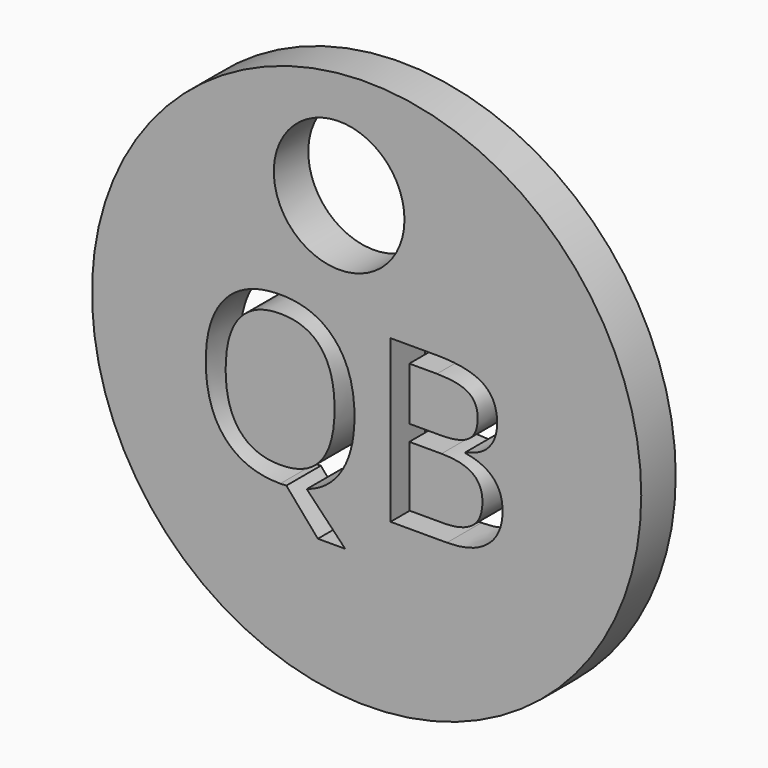
from build123d import *

# Parameters (mm, degrees)
F0_R         = 13.7039502502
F1_DEPTH     = 2.15
F2_R         = 3.2599586052
F3_DEPTH     = 2.15
F4_TEXT_SIZE = 11.3007392631
F5_DEPTH     = 2.15


# Not quite as in the source:
# - Text() gives the source's letters only with a copy of the font that has no kerning and outlines rounded to 1/6400 em; it was checked with that copy


with BuildPart() as f1:
    # F0 (on Front) → F1 (new body)
    with BuildSketch(Plane.XZ):
        with Locations((-43.4432663023, -15.2559969574)):
            Circle(F0_R)
    extrude(amount=F1_DEPTH)

    # F2 (on Front) → F3 (cut, through all)
    with BuildSketch(Plane.XZ):
        with Locations((-44.8150597513, -6.9880178198)):
            Circle(F2_R)
    extrude(amount=F3_DEPTH, mode=Mode.SUBTRACT)

    # F4 (on Front) → F5 (cut, through all)
    with BuildSketch(Plane.XZ):
        with Locations((-52.1609783173, -20.4866249114)):
            Text('QB', F4_TEXT_SIZE, font='Open Sans', text_align=(TextAlign.LEFT, TextAlign.BOTTOM))
    extrude(amount=F5_DEPTH, mode=Mode.SUBTRACT)


solid = f1.part
